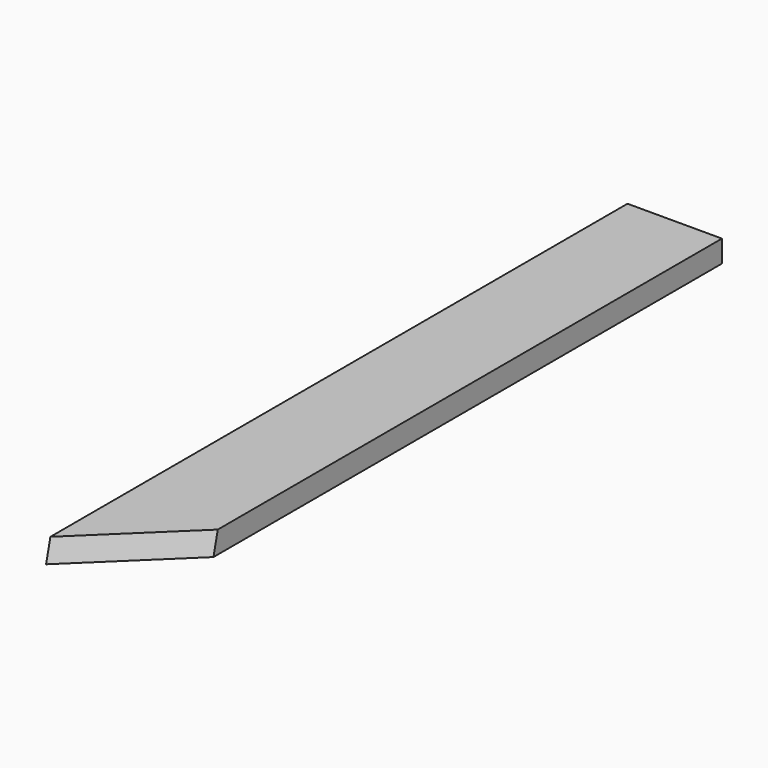
from build123d import *

# Parameters (mm, degrees)
F0_W        = 120
F0_H        = 28
F1_DEPTH    = 462.5
F2_SIZE2    = 115.882643
F2_SIZE     = 119.99999
F3_T1_DEPTH = 343.6641668027


# Not quite as in the source:
# - a fillet or chamfer that OpenCascade refuses, or shapes differently, is made with other operations: its cross-section is extruded or revolved along the edge and cut away or added
# - a fillet or chamfer is up to 0.001 mm smaller than in the source, because OpenCascade refuses the exact size


with BuildPart() as f1:
    # F0 (on Front) → F1 (new body, symmetric)
    with BuildSketch(Plane.XZ):
        Rectangle(F0_W, F0_H)
    extrude(amount=F1_DEPTH, both=True)

    # F2 (size 120 and 115.8826529768 in the source; OpenCascade refuses exactly that, so slightly less here)
    f2_edges = [f1.edges().sort_by_distance(p)[0] for p in [
        (60, -462.5, 0),
    ]]
    f2_side = f1.faces().sort_by_distance((0, -462.5, 0))[0]
    chamfer(f2_edges, length=F2_SIZE, length2=F2_SIZE2, reference=f2_side)

    # F3: chamfer of 6 x 34.0276909177 on 2 edges, made by hand

    # F3_s2 → F3_t1 (cut)
    with BuildSketch(Plane(origin=(-325.7617702656, -314.5844839382, 0), x_dir=(0, 0, 1), z_dir=(0.7193398013, 0.6946583695, 0))):
        Polygon((-20.0276909177, 291.0151628785), (14, 285.0151628785), (14, 291.0151628785), align=None)
    extrude(amount=F3_T1_DEPTH, mode=Mode.SUBTRACT)


solid = f1.part
